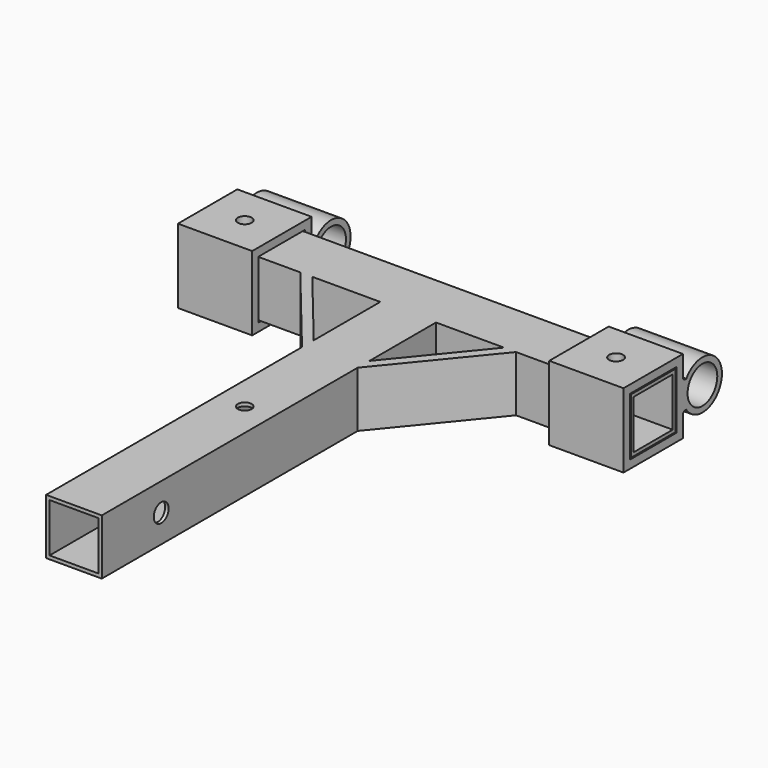
from build123d import *

# Parameters (mm, degrees)
F0_W      = 38.1
F0_H      = 38.1
F0_W_2    = 33.3375
F0_H_2    = 33.3375
F1_DEPTH  = 304.8
F2_W      = 38.1
F2_H      = 38.1
F2_W_2    = 33.3375
F2_H_2    = 33.3375
F3_DEPTH  = 304.8
F4_W      = 39.6875
F4_H      = 39.6875
F4_R      = 12.7
F5_DEPTH  = 50.8
F7_R      = 4.7625
F8_DEPTH  = 50.801
F9_R      = 4.7625
F10_DEPTH = 50.801
F11_R     = 6.35
F12_DEPTH = 171.451
F15_DEPTH = 38.1
F16_R     = 4.7625
F17_DEPTH = 44.451


# Not quite as in the source:
# - a pattern or mirror of a feature is missing from the dataset's text; its kind, count and spacing are read off the source's solid
# - a feature names something its author has since deleted; it is built from what else it names


with BuildPart() as f1:
    # F0 (on Right) → F1 (new body)
    with BuildSketch(Plane.YZ):
        Rectangle(F0_W, F0_H)
        Rectangle(F0_W_2, F0_H_2, mode=Mode.SUBTRACT)
    extrude(amount=-F1_DEPTH)

    # F2 (on Front) → F3 (join)
    with BuildSketch(Plane.XZ):
        with Locations((-152.4, 0)):
            Rectangle(F2_W, F2_H)
        with Locations((-152.4, 0)):
            Rectangle(F2_W_2, F2_H_2, mode=Mode.SUBTRACT)
    extrude(amount=F3_DEPTH)


with BuildPart() as f5:
    # F4 (on Right) → F5 (new body)
    with BuildSketch(Plane.YZ):
        Polygon((25.4, 10.626129806), (25.4, 25.4), (-25.4, 25.4), (-25.4, -25.4), (25.4, -25.4), (25.4, -10.626129806), (25.4, -1.82e-08), align=None)
        Rectangle(F4_W, F4_H, mode=Mode.SUBTRACT)
        with BuildLine():
            ThreePointArc((28.2387536196, 9.3047529082), (26.5696544388, 9.428955298), (25.4, 10.626129806))
            Line((25.4, 10.626129806), (25.4, -1.82e-08))
            ThreePointArc((25.4, -1.82e-08), (26.1254758868, 4.864076183), (28.2387536196, 9.3047529082))
        make_face()
        with BuildLine():
            ThreePointArc((28.2387536196, -9.3047529082), (26.1254758921, -4.8640762004), (25.4, -1.82e-08))
            Line((25.4, -1.82e-08), (25.4, -10.626129806))
            ThreePointArc((25.4, -10.626129806), (26.5696544388, -9.428955298), (28.2387536196, -9.3047529082))
        make_face()
        with BuildLine():
            ThreePointArc((28.2387536196, 9.3047529082), (26.1254758868, 4.864076183), (25.4, -1.82e-08))
            ThreePointArc((25.4, -1.82e-08), (26.1254758921, -4.8640762004), (28.2387536196, -9.3047529082))
            ThreePointArc((28.2387536196, -9.3047529082), (46.9328261917, -15.9432741105), (58.7375, 0))
            ThreePointArc((58.7375, 0), (46.9328261917, 15.9432741105), (28.2387536196, 9.3047529082))
        make_face()
        with Locations((42.06875, 0)):
            Circle(F4_R, mode=Mode.SUBTRACT)
    extrude(amount=-F5_DEPTH)


with BuildPart() as f6_1:
    # F6: copy of F5
    add(f5.part.moved(Location((-254, 0, 0))))


with BuildPart() as f8_tool:
    # F7 (on face) → F8 (new body, through all)
    with BuildSketch(Plane.XY.offset(25.4)):
        with Locations((-25.4, 0)):
            Circle(F7_R)
    extrude(amount=-F8_DEPTH)


with BuildPart() as f1_1:
    add(f1.part)

    # F8: cut by f8_tool
    add(f8_tool.part, mode=Mode.SUBTRACT)


with BuildPart() as f5_1:
    add(f5.part)

    # F8: cut by f8_tool
    add(f8_tool.part, mode=Mode.SUBTRACT)


with BuildPart() as f10_tool:
    # F9 (on face) → F10 (new body, through all)
    with BuildSketch(Plane.XY.offset(25.4)):
        with Locations((-279.4, 0)):
            Circle(F9_R)
    extrude(amount=-F10_DEPTH)


with BuildPart() as f1_2:
    add(f1_1.part)

    # F10: cut by f10_tool
    add(f10_tool.part, mode=Mode.SUBTRACT)

    # F11 (on face) → F12 (cut, through all)
    with BuildSketch(Plane.YZ.offset(-133.35)):
        with Locations((-254, 0)):
            Circle(F11_R)
    extrude(amount=-F12_DEPTH, mode=Mode.SUBTRACT)

    # F13 (on face) → F15 (join)
    with BuildSketch(Plane.XY.offset(19.05)):
        Polygon((-78.6219015718, -19.05), (-86.8246659974, -19.05), (-133.35, -75.9458216504), (-133.35, -85.9769806266), align=None)
    f15 = extrude(amount=-F15_DEPTH)

    # F15_copies: F15 across plane
    add(f15.mirror(Plane(origin=(-152.4, 0, 0), x_dir=(0, 0, -1), z_dir=(-1, 0, 0))))

    # F16 (on face) → F17 (cut, through all)
    with BuildSketch(Plane.XY.offset(19.05)):
        with Locations((-152.4, -158.75)):
            Circle(F16_R)
    extrude(amount=-F17_DEPTH, mode=Mode.SUBTRACT)


with BuildPart() as f6_1_1:
    add(f6_1.part)

    # F10: cut by f10_tool
    add(f10_tool.part, mode=Mode.SUBTRACT)


solid = Compound([f5_1.part, f1_2.part, f6_1_1.part])
